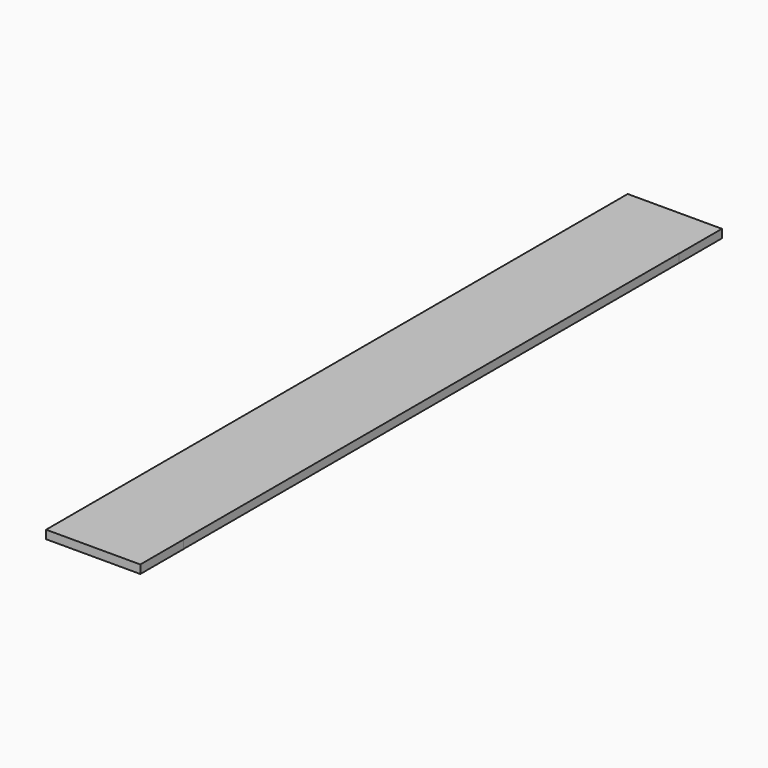
from build123d import *

# Parameters (mm, degrees)
F0_W     = 118.618
F0_H     = 2336.8
F0_W_2   = 118.364
F1_DEPTH = 31.75


# Not quite as in the source:
# - a feature names something its author has since deleted; it is built from what else it names


with BuildPart() as f1:
    # F0 (on Top) → F1 (new body)
    with BuildSketch(Plane.XY):
        Polygon((-49.4727902114, 129.2092303157), (-49.4727902114, -73.9907696843), (306.1272097886, -73.9907696843), (306.1272097886, 129.2092303157), (305.8732097886, 129.2092303157), (187.2552097886, 129.2092303157), (68.8912097886, 129.2092303157), align=None)
        with Locations((246.5642097886, 1297.6092303157)):
            Rectangle(F0_W, F0_H)
        with Locations((128.0732097886, 1297.6092303157)):
            Rectangle(F0_W_2, F0_H)
        with Locations((9.7092097886, 1297.6092303157)):
            Rectangle(F0_W_2, F0_H)
        Polygon((-49.4727902114, 2669.2092303157), (-49.4727902114, 2466.0092303157), (68.8912097886, 2466.0092303157), (187.2552097886, 2466.0092303157), (305.8732097886, 2466.0092303157), (306.1272097886, 2466.0092303157), (306.1272097886, 2669.2092303157), align=None)
    extrude(amount=F1_DEPTH)


solid = f1.part
